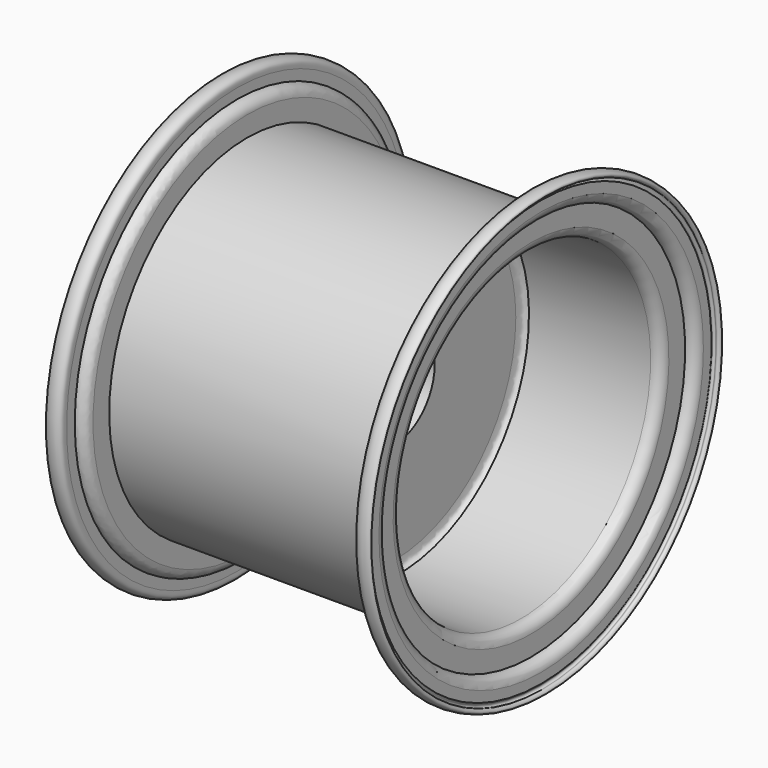
from build123d import *

# Parameters (mm, degrees)
F2_R     = 10
F3_DEPTH = 20
F4_COUNT = 6
F4_ANGLE = 1800


with BuildPart() as f1:
    # F0 (on Front) → F1 (revolve)
    with BuildSketch(Plane.XZ):
        with BuildLine():
            Line((-135, 160), (-15, 160))
            add(Edge.make_bspline(
                [(-15, 160), (-9.7317537293, 157.3773622513), (-10.0691160187, 153.4736007452), (-10, 150)],
                knots=[0, 0, 0, 0, 11.1803398875, 11.1803398875, 11.1803398875, 11.1803398875], degree=3))
            Line((-10, 150), (-10, 50))
            Line((-10, 50), (10, 50))
            Line((10, 50), (10, 150))
            add(Edge.make_bspline(
                [(15, 160), (9.7317537293, 157.3773622513), (10.0691160187, 153.4736007452), (10, 150)],
                knots=[0, 0, 0, 0, 11.1803398875, 11.1803398875, 11.1803398875, 11.1803398875], degree=3))
            Line((15, 160), (135, 160))
            ThreePointArc((135, 160), (142.0710678119, 162.9289321881), (145, 170))
            Line((145, 170), (145, 190))
            ThreePointArc((145, 190), (152.0710678119, 192.9289321881), (155, 200))
            Line((155, 200), (155, 210))
            add(Edge.make_bspline(
                [(155, 210), (154.1086140007, 211.1240821505), (152.3350454635, 213.2323719114), (155.1753279482, 215.9921208461), (157.3405565473, 212.3275316174), (161.811688282, 217.1360260026), (155.0984836266, 219.6086922807), (148.8577992246, 219.2225416492), (144.5157139111, 216.1587826782), (144.8595434531, 212.0745483949), (145, 210)],
                knots=[0, 0, 0, 0, 0.1185623844, 0.2114002837, 0.3132307231, 0.4301321809, 0.5684633303, 0.7250232514, 0.8534984859, 1, 1, 1, 1], degree=3))
            Line((145, 210), (145, 200))
            add(Edge.make_bspline(
                [(145, 200), (140.7763447651, 200.1355448859), (134.836930118, 196.3598314841), (135, 189.9961233139)],
                knots=[0, 0, 0, 0, 14.1448771204, 14.1448771204, 14.1448771204, 14.1448771204], degree=3))
            Line((135, 189.9961233139), (135, 170))
            Line((135, 170), (-135, 170))
            Line((-135, 170), (-135, 189.9961233139))
            add(Edge.make_bspline(
                [(-145, 200), (-140.7763447651, 200.1355448859), (-134.836930118, 196.3598314841), (-135, 189.9961233139)],
                knots=[0, 0, 0, 0, 14.1448771204, 14.1448771204, 14.1448771204, 14.1448771204], degree=3))
            Line((-145, 200), (-145, 210))
            add(Edge.make_bspline(
                [(-155, 210), (-154.1086140007, 211.1240821505), (-152.3350454635, 213.2323719114), (-155.1753279482, 215.9921208461), (-157.3405565473, 212.3275316174), (-161.811688282, 217.1360260026), (-155.0984836266, 219.6086922807), (-148.8577992246, 219.2225416492), (-144.5157139111, 216.1587826782), (-144.8595434531, 212.0745483949), (-145, 210)],
                knots=[0, 0, 0, 0, 0.1185623844, 0.2114002837, 0.3132307231, 0.4301321809, 0.5684633303, 0.7250232514, 0.8534984859, 1, 1, 1, 1], degree=3))
            Line((-155, 210), (-155, 200))
            ThreePointArc((-155, 200), (-152.0710678119, 192.9289321881), (-145, 190))
            Line((-145, 190), (-145, 170))
            ThreePointArc((-145, 170), (-142.0710678119, 162.9289321881), (-135, 160))
        make_face()
    revolve(axis=Axis((-3.6142840981, 0, 0), (1, 0, 0)))

    # F2 (on face) → F3 (cut)
    with BuildSketch(Plane.YZ.offset(10)):
        with Locations((0, 80)):
            Circle(F2_R)
    extrude(amount=-F3_DEPTH, mode=Mode.SUBTRACT)

    # F4: F1 ×6 about axis
    f4_axis = Axis((-3.6142840981, 0, 0), (-1, 0, 0))


with BuildPart() as f1_1:
    add(f1.part)
    for i in range(1, F4_COUNT):
        add(f1.part.rotate(f4_axis, i * F4_ANGLE / (F4_COUNT - 1)))


solid = f1_1.part
